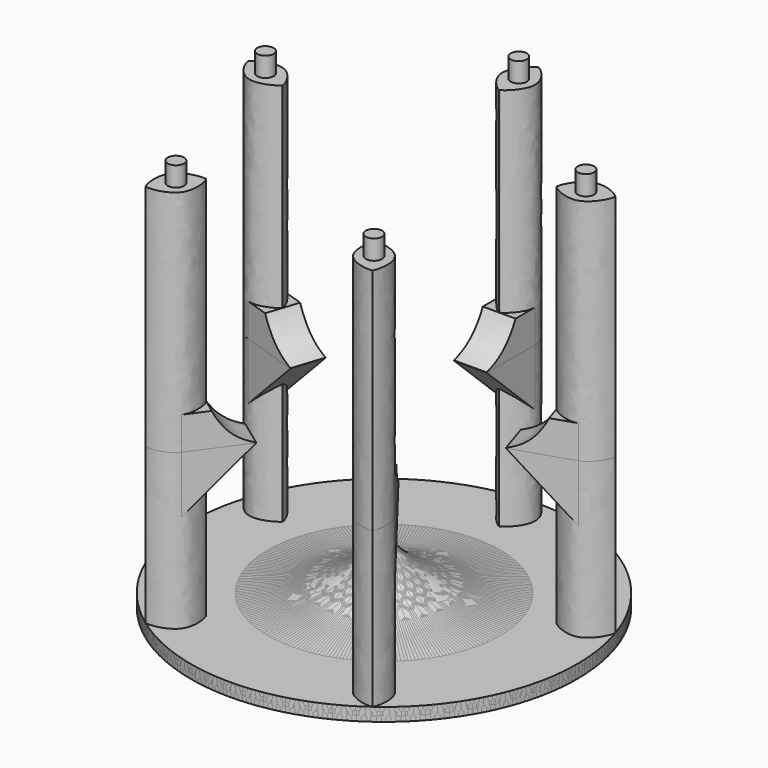
from build123d import *

# Parameters (mm, degrees)
F0_R      = 59
F0_R_2    = 44
F1_DEPTH  = 4.03
F3_DEPTH  = 47.41
F5_DEPTH  = 0.1
F7_DEPTH  = 10
F9_DEPTH  = 10
F11_DEPTH = 70
F12_R     = 2.5
F13_DEPTH = 6
F16_COUNT = 5


with BuildPart() as f1:
    # F0 (on Top) → F1 (new body)
    with BuildSketch(Plane.XY):
        Circle(F0_R)
        Circle(F0_R_2, mode=Mode.SUBTRACT)
        Circle(F0_R_2)
    extrude(amount=F1_DEPTH)

    # F2 (on face) → F3 (join)
    with BuildSketch(Plane.XY.offset(4.03)):
        with BuildLine():
            add(Edge.make_bspline(
                [(5, 51.5), (5, 48.05), (1.5, 44.6), (0, 44)],
                knots=[0.5, 0.5, 0.5, 0.5, 1, 1, 1, 1], degree=3))
            Line((5, 51.5), (-5, 51.5))
            add(Edge.make_bspline(
                [(0, 44), (-1.5, 44.6), (-5, 48.05), (-5, 51.5)],
                knots=[0, 0, 0, 0, 0.5, 0.5, 0.5, 0.5], degree=3))
        make_face()
        with BuildLine():
            add(Edge.make_bspline(
                [(0, 59), (1.5, 58.4), (5, 54.95), (5, 51.5)],
                knots=[0, 0, 0, 0, 0.5, 0.5, 0.5, 0.5], degree=3))
            add(Edge.make_bspline(
                [(-5, 51.5), (-5, 54.95), (-1.5, 58.4), (0, 59)],
                knots=[0.5, 0.5, 0.5, 0.5, 1, 1, 1, 1], degree=3))
            Line((-5, 51.5), (5, 51.5))
        make_face()
    extrude(amount=F3_DEPTH)

    # F4 (on face) → F5 (join)
    with BuildSketch(Plane.XY.offset(51.44)):
        with BuildLine():
            ThreePointArc((5, 43.7149859888), (2.5040583553, 43.9286887097), (0, 44))
            ThreePointArc((0, 44), (-2.5040583553, 43.9286887097), (-5, 43.7149859888))
            Line((-5, 43.7149859888), (-5, 33))
            Line((-5, 33), (5, 33))
            Line((5, 33), (5, 43.7149859888))
        make_face()
        with BuildLine():
            Line((5, 43.7149859888), (5, 51.5))
            add(Edge.make_bspline(
                [(5, 51.5), (5, 48.05), (1.5, 44.6), (0, 44)],
                knots=[0.5, 0.5, 0.5, 0.5, 1, 1, 1, 1], degree=3))
            ThreePointArc((0, 44), (2.5040583553, 43.9286887097), (5, 43.7149859888))
        make_face()
        with BuildLine():
            add(Edge.make_bspline(
                [(0, 44), (-1.5, 44.6), (-5, 48.05), (-5, 51.5)],
                knots=[0, 0, 0, 0, 0.5, 0.5, 0.5, 0.5], degree=3))
            Line((-5, 51.5), (-5, 43.7149859888))
            ThreePointArc((-5, 43.7149859888), (-2.5040583553, 43.9286887097), (0, 44))
        make_face()
    extrude(amount=F5_DEPTH)

    # F8 (on face) → F9 (join)
    with BuildSketch(Plane(origin=(-5, 0, 0), x_dir=(0, -1, 0), z_dir=(-1, 0, 0))):
        with BuildLine():
            Line((-44, 61.54), (-51.5, 61.54))
            Line((-51.5, 61.54), (-51.5, 51.54))
            Line((-51.5, 51.54), (-33, 51.54))
            add(Edge.make_bspline(
                [(-44, 61.54), (-43.5887060934, 60.5884753951), (-42.6630172378, 58.908110353), (-40.2992639723, 55.670403168), (-36.9929729635, 53.0551214475), (-34.3587183904, 52.0116398107), (-33, 51.54)],
                knots=[0, 0, 0, 0, 0.2200073166, 0.4735064445, 0.7359247823, 1, 1, 1, 1], degree=3))
        make_face()
    extrude(amount=-F9_DEPTH)

    # F14 (on Right) → F15 (revolve)
    with BuildSketch(Plane.YZ):
        with BuildLine():
            Line((0, 21.45), (0, 4.03))
            Line((0, 4.03), (35.5, 4.03))
            add(Edge.make_bspline(
                [(35.5, 4.03), (31.0577831602, 4.5559429128), (26.8296379483, 4.8318487951), (18.3648538576, 6.2293134194), (12.0234292715, 9.333070349), (6.7765394638, 12.4664569508), (2.1705765265, 17.0114363048), (0.6305386362, 19.7930387028), (0, 21.45)],
                knots=[0, 0, 0, 0, 0.1943631818, 0.3727819007, 0.5418584521, 0.6995198485, 0.8585493006, 1, 1, 1, 1], degree=3))
        make_face()
    revolve(axis=Axis((0, 0, 0), (0, 0, -1)))


with BuildPart() as f7:
    # F6 (on face) → F7 (new body)
    with BuildSketch(Plane(origin=(-5, 0, 0), x_dir=(0, -1, 0), z_dir=(-1, 0, 0))):
        Polygon((-33, 51.44), (-51.5, 51.44), (-51.5, 33.9189), align=None)
    extrude(amount=-F7_DEPTH)


with BuildPart() as f11:
    # F10 (on face) → F11 (new body)
    with BuildSketch(Plane.XY.offset(51.44)):
        with BuildLine():
            add(Edge.make_bspline(
                [(0.2151426403, 44.0985608791), (0.1358182805, 44.0584926842), (0.0638343199, 44.0255337279), (0, 44)],
                knots=[0.9787218934, 0.9787218934, 0.9787218934, 0.9787218934, 1, 1, 1, 1], degree=3))
            add(Edge.make_bspline(
                [(0.2151426403, 44.0985608791), (1.8092390852, 44.9118693925), (5, 48.2059346962), (5, 51.5)],
                knots=[0.5225992313, 0.5225992313, 0.5225992313, 0.5225992313, 1, 1, 1, 1], degree=3))
            add(Edge.make_bspline(
                [(5, 51.5), (5, 54.95), (1.5, 58.4), (0, 59)],
                knots=[1, 1, 1, 1, 1.5, 1.5, 1.5, 1.5], degree=3))
            add(Edge.make_bspline(
                [(0, 59), (-1.5, 58.4), (-5, 54.95), (-5, 51.5)],
                knots=[0.5, 0.5, 0.5, 0.5, 1, 1, 1, 1], degree=3))
            add(Edge.make_bspline(
                [(-5, 51.5), (-5, 48.2059346962), (-1.8092390852, 44.9118693925), (-0.2151426403, 44.0985608791)],
                knots=[1, 1, 1, 1, 1.4774007687, 1.4774007687, 1.4774007687, 1.4774007687], degree=3))
            add(Edge.make_bspline(
                [(0, 44), (-0.0638343199, 44.0255337279), (-0.1358182805, 44.0584926842), (-0.2151426403, 44.0985608791)],
                knots=[0, 0, 0, 0, 0.0212781066, 0.0212781066, 0.0212781066, 0.0212781066], degree=3))
        make_face()
    extrude(amount=F11_DEPTH)


with BuildPart() as f13:
    # F12 (on face) → F13 (new body)
    with BuildSketch(Plane.XY.offset(121.44)):
        with Locations((0, 51.5)):
            Circle(F12_R)
    extrude(amount=F13_DEPTH)


with BuildPart() as f16_1:
    # F16: instance of F1
    add(f1.part.rotate(Axis((0, 0, 0), (0, 0, 1)), 1 * 360 / F16_COUNT))


with BuildPart() as f16_2:
    # F16: instance of F1
    add(f1.part.rotate(Axis((0, 0, 0), (0, 0, 1)), 2 * 360 / F16_COUNT))


with BuildPart() as f16_3:
    # F16: instance of F1
    add(f1.part.rotate(Axis((0, 0, 0), (0, 0, 1)), 3 * 360 / F16_COUNT))


with BuildPart() as f16_4:
    # F16: instance of F1
    add(f1.part.rotate(Axis((0, 0, 0), (0, 0, 1)), 4 * 360 / F16_COUNT))


with BuildPart() as f16_5:
    # F16: instance of F7
    add(f7.part.rotate(Axis((0, 0, 0), (0, 0, 1)), 1 * 360 / F16_COUNT))


with BuildPart() as f16_6:
    # F16: instance of F7
    add(f7.part.rotate(Axis((0, 0, 0), (0, 0, 1)), 2 * 360 / F16_COUNT))


with BuildPart() as f16_7:
    # F16: instance of F7
    add(f7.part.rotate(Axis((0, 0, 0), (0, 0, 1)), 3 * 360 / F16_COUNT))


with BuildPart() as f16_8:
    # F16: instance of F7
    add(f7.part.rotate(Axis((0, 0, 0), (0, 0, 1)), 4 * 360 / F16_COUNT))


with BuildPart() as f16_9:
    # F16: instance of F11
    add(f11.part.rotate(Axis((0, 0, 0), (0, 0, 1)), 1 * 360 / F16_COUNT))


with BuildPart() as f16_10:
    # F16: instance of F11
    add(f11.part.rotate(Axis((0, 0, 0), (0, 0, 1)), 2 * 360 / F16_COUNT))


with BuildPart() as f16_11:
    # F16: instance of F11
    add(f11.part.rotate(Axis((0, 0, 0), (0, 0, 1)), 3 * 360 / F16_COUNT))


with BuildPart() as f16_12:
    # F16: instance of F11
    add(f11.part.rotate(Axis((0, 0, 0), (0, 0, 1)), 4 * 360 / F16_COUNT))


with BuildPart() as f16_13:
    # F16: instance of F13
    add(f13.part.rotate(Axis((0, 0, 0), (0, 0, 1)), 1 * 360 / F16_COUNT))


with BuildPart() as f16_14:
    # F16: instance of F13
    add(f13.part.rotate(Axis((0, 0, 0), (0, 0, 1)), 2 * 360 / F16_COUNT))


with BuildPart() as f16_15:
    # F16: instance of F13
    add(f13.part.rotate(Axis((0, 0, 0), (0, 0, 1)), 3 * 360 / F16_COUNT))


with BuildPart() as f16_16:
    # F16: instance of F13
    add(f13.part.rotate(Axis((0, 0, 0), (0, 0, 1)), 4 * 360 / F16_COUNT))


solid = Compound([f1.part, f7.part, f11.part, f13.part, f16_1.part, f16_2.part, f16_3.part, f16_4.part, f16_5.part, f16_6.part, f16_7.part, f16_8.part, f16_9.part, f16_10.part, f16_11.part, f16_12.part, f16_13.part, f16_14.part, f16_15.part, f16_16.part])
